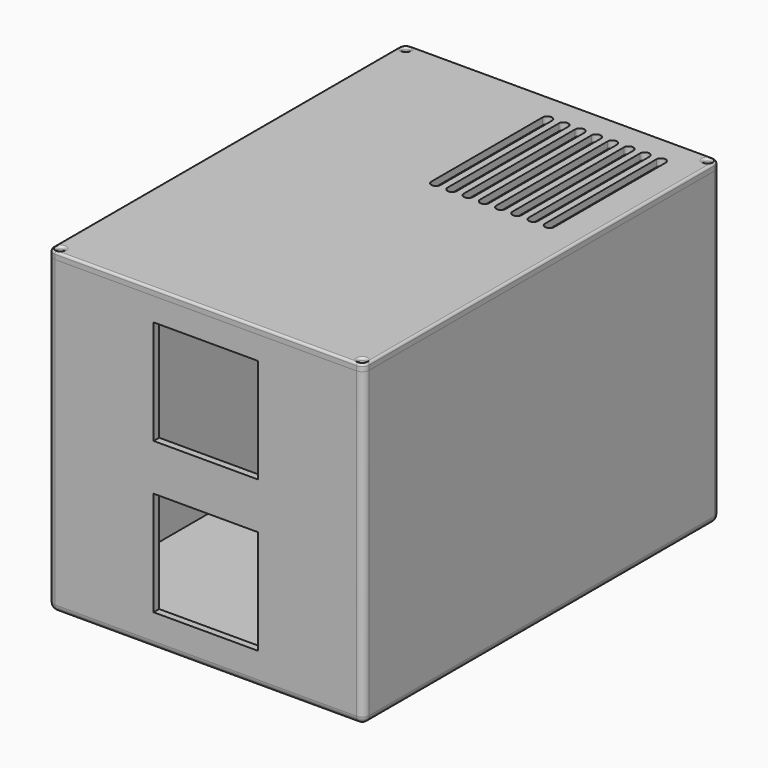
from build123d import *

# Parameters (mm, degrees)
F0_W          = 136
F0_H          = 192
F1_DEPTH      = 4
F2_DEPTH      = 134
F3_W          = 45
F3_H          = 45
F4_DEPTH      = 25
F5_W          = 84
F5_H          = 10
F6_DEPTH      = 20
F8_DEPTH      = 10
F9_W          = 10
F9_H          = 107
F9_R          = 1.5
F10_DEPTH     = 15
F11_R         = 1.5
F12_DEPTH     = 10
F13_W         = 10
F13_H         = 10
F13_W_2       = 27
F13_H_2       = 66
F13_H_3       = 19
F13_R         = 1.6
F14_DEPTH     = 25
F15_W         = 27
F15_H         = 7.5
F16_DEPTH     = 1.5
F17_SIZE      = 1.49999
F18_R         = 3
F19_R         = 3
F20_R         = 3
F22_W         = 65
F22_H         = 125
F22_W_2       = 45
F22_H_2       = 45
F23_DEPTH     = 10
F24_SIZE      = 1
F26_R         = 1.5
F27_DEPTH     = 3
F28_T1_DEPTH  = 186
F28_T3_DEPTH  = 130
F28_T6_ANGLE  = 90
F28_T8_ANGLE  = 90
F28_T10_ANGLE = 90
F28_T12_ANGLE = 90
F30_DEPTH     = 25


# Not quite as in the source:
# - a fillet or chamfer that OpenCascade refuses, or shapes differently, is made with other operations: its cross-section is extruded or revolved along the edge and cut away or added
# - a fillet or chamfer is up to 0.001 mm smaller than in the source, because OpenCascade refuses the exact size


with BuildPart() as f1:
    # F0 (on Top) → F1 (new body)
    with BuildSketch(Plane.XY):
        Rectangle(F0_W, F0_H)
        with BuildLine():
            ThreePointArc((65, -88), (61.4644660941, -89.4644660941), (60, -93))
            Line((60, -93), (-60, -93))
            ThreePointArc((-60, -93), (-61.4644660941, -89.4644660941), (-65, -88))
            Line((-65, -88), (-65, 88))
            ThreePointArc((-65, 88), (-61.4644660941, 89.4644660941), (-60, 93))
            Line((-60, 93), (60, 93))
            ThreePointArc((60, 93), (61.4644660941, 89.4644660941), (65, 88))
            Line((65, 88), (65, -88))
        make_face(mode=Mode.SUBTRACT)
        with BuildLine():
            Line((-60, -93), (60, -93))
            ThreePointArc((60, -93), (61.4644660941, -89.4644660941), (65, -88))
            Line((65, -88), (65, 88))
            ThreePointArc((65, 88), (61.4644660941, 89.4644660941), (60, 93))
            Line((60, 93), (-60, 93))
            ThreePointArc((-60, 93), (-61.4644660941, 89.4644660941), (-65, 88))
            Line((-65, 88), (-65, -88))
            ThreePointArc((-65, -88), (-61.4644660941, -89.4644660941), (-60, -93))
        make_face()
    extrude(amount=F1_DEPTH)

    # F0 (on Top) → F2 (join)
    with BuildSketch(Plane.XY):
        Rectangle(F0_W, F0_H)
        with BuildLine():
            ThreePointArc((65, -88), (61.4644660941, -89.4644660941), (60, -93))
            Line((60, -93), (-60, -93))
            ThreePointArc((-60, -93), (-61.4644660941, -89.4644660941), (-65, -88))
            Line((-65, -88), (-65, 88))
            ThreePointArc((-65, 88), (-61.4644660941, 89.4644660941), (-60, 93))
            Line((-60, 93), (60, 93))
            ThreePointArc((60, 93), (61.4644660941, 89.4644660941), (65, 88))
            Line((65, 88), (65, -88))
        make_face(mode=Mode.SUBTRACT)
    extrude(amount=F2_DEPTH)

    # F3 (on face) → F4 (cut)
    with BuildSketch(Plane.XZ.offset(96)):
        with Locations((0, 101.5)):
            Rectangle(F3_W, F3_H)
        with Locations((0, 36.5)):
            Rectangle(F3_W, F3_H)
    extrude(amount=-F4_DEPTH, mode=Mode.SUBTRACT)

    # F5 (on face) → F6 (join)
    with BuildSketch(Plane.XY.offset(4)):
        with Locations((-23, 78)):
            Rectangle(F5_W, F5_H)
    extrude(amount=F6_DEPTH)

    # F7 (on face) → F8 (cut)
    with BuildSketch(Plane.XZ.offset(-73)):
        Polygon((9, 24), (19, 24), (19, 33.6412377656), (-55, 33.6412377656), (-55, 14), (-28, 14), (-28, 24), (-18, 24), (-18, 14), (9, 14), align=None)
    extrude(amount=-F8_DEPTH, mode=Mode.SUBTRACT)

    # F9 (on face) → F10 (join)
    with BuildSketch(Plane(origin=(65, 0, 0), x_dir=(0, -1, 0), z_dir=(-1, 0, 0))):
        with Locations((-78, 57.5)):
            Rectangle(F9_W, F9_H)
        with Locations((-78, 19)):
            Circle(F9_R, mode=Mode.SUBTRACT)
        with Locations((-78, 106)):
            Circle(F9_R, mode=Mode.SUBTRACT)
        with Locations((-24, 57.5)):
            Rectangle(F9_W, F9_H)
        with Locations((-24, 19)):
            Circle(F9_R, mode=Mode.SUBTRACT)
        with Locations((-24, 106)):
            Circle(F9_R, mode=Mode.SUBTRACT)
    extrude(amount=F10_DEPTH)

    # F11 (on face) → F12 (cut)
    with BuildSketch(Plane.XY.offset(134)):
        with Locations((65, 93)):
            Circle(F11_R)
        with Locations((-65, 93)):
            Circle(F11_R)
        with Locations((65, -93)):
            Circle(F11_R)
        with Locations((-65, -93)):
            Circle(F11_R)
    extrude(amount=-F12_DEPTH, mode=Mode.SUBTRACT)

    # F13 (on face) → F14 (cut)
    with BuildSketch(Plane(origin=(0, 96, 0), x_dir=(-1, 0, 0), z_dir=(0, 1, 0))):
        with Locations((-40, 129)):
            Rectangle(F13_W, F13_H)
        with Locations((41.5, 47)):
            Rectangle(F13_W_2, F13_H_2)
        with Locations((4.5, 47)):
            Rectangle(F13_W_2, F13_H_2)
        with Locations((-24, 26.5)):
            Rectangle(F13_W, F13_H_3)
        with Locations((-24, 14)):
            Circle(F13_R)
        with Locations((-24, 39)):
            Circle(F13_R)
        with Locations((-24, 49)):
            Circle(F13_R)
        with Locations((-24, 61.5)):
            Rectangle(F13_W, F13_H_3)
        with Locations((-24, 74)):
            Circle(F13_R)
    extrude(amount=-F14_DEPTH, mode=Mode.SUBTRACT)

    # F15 (on face) → F16 (cut)
    with BuildSketch(Plane.XZ.offset(-93)):
        with Locations((-41.5, 83.75)):
            Rectangle(F15_W, F15_H)
        with Locations((-4.5, 83.75)):
            Rectangle(F15_W, F15_H)
        with Locations((-41.5, 10.25)):
            Rectangle(F15_W, F15_H)
        with Locations((-4.5, 10.25)):
            Rectangle(F15_W, F15_H)
    extrude(amount=-F16_DEPTH, mode=Mode.SUBTRACT)

    # F17 (size 1.5 in the source; OpenCascade refuses exactly that, so slightly less here)
    f17_edges = [f1.edges().sort_by_distance(p)[0] for p in [
        (-4.5, 94.5, 6.5),
        (-41.5, 94.5, 6.5),
        (-4.5, 94.5, 87.5),
        (-41.5, 94.5, 87.5),
    ]]
    chamfer(f17_edges, length=F17_SIZE)

    # F18
    f18_edges = [f1.edges().sort_by_distance(p)[0] for p in [
        (-68, -96, 67),
        (68, -96, 67),
        (68, 96, 67),
        (-68, 96, 67),
    ]]
    fillet(f18_edges, radius=F18_R)

    # F19
    f19_edges = [f1.edges().sort_by_distance(p)[0] for p in [
        (0, -96, 0),
    ]]
    fillet(f19_edges, radius=F19_R)

    # F20
    f20_edges = [f1.edges().sort_by_distance(p)[0] for p in [
        (45, 94.5, 124),
        (35, 94.5, 124),
    ]]
    fillet(f20_edges, radius=F20_R)


with BuildPart() as f23:
    # F22 (on offset) → F23 (new body)
    with BuildSketch(Plane(origin=(0, -23, 0), x_dir=(-1, 0, 0), z_dir=(0, 1, 0))):
        with Locations((0, 66.5)):
            Rectangle(F22_W, F22_H)
        with Locations((0, 36.5)):
            Rectangle(F22_W_2, F22_H_2, mode=Mode.SUBTRACT)
        with Locations((0, 101.5)):
            Rectangle(F22_W_2, F22_H_2, mode=Mode.SUBTRACT)
    extrude(amount=F23_DEPTH)

    # F24
    f24_edges = [f23.edges().sort_by_distance(p)[0] for p in [
        (-32.5, -23, 66.5),
        (0, -23, 129),
        (32.5, -23, 66.5),
        (0, -23, 4),
        (22.5, -23, 36.5),
        (0, -23, 59),
        (-22.5, -23, 36.5),
        (0, -23, 14),
        (22.5, -23, 101.5),
        (0, -23, 124),
        (-22.5, -23, 101.5),
        (0, -23, 79),
        (-32.5, -13, 66.5),
        (0, -13, 129),
        (32.5, -13, 66.5),
        (0, -13, 4),
        (22.5, -13, 36.5),
        (0, -13, 59),
        (-22.5, -13, 36.5),
        (0, -13, 14),
        (22.5, -13, 101.5),
        (0, -13, 124),
        (-22.5, -13, 101.5),
        (0, -13, 79),
    ]]
    chamfer(f24_edges, length=F24_SIZE)


with BuildPart() as f27:
    # F26 (on offset) → F27 (new body)
    with BuildSketch(Plane.XY.offset(134)):
        with BuildLine():
            ThreePointArc((65, -96), (67.1213203436, -95.1213203436), (68, -93))
            Line((68, -93), (68, 93))
            ThreePointArc((68, 93), (67.1213203436, 95.1213203436), (65, 96))
            Line((65, 96), (-65, 96))
            ThreePointArc((-65, 96), (-67.1213203436, 95.1213203436), (-68, 93))
            Line((-68, 93), (-68, -93))
            ThreePointArc((-68, -93), (-67.1213203436, -95.1213203436), (-65, -96))
            Line((-65, -96), (65, -96))
        make_face()
        with Locations((-65, -93)):
            Circle(F26_R, mode=Mode.SUBTRACT)
        with Locations((65, -93)):
            Circle(F26_R, mode=Mode.SUBTRACT)
        with Locations((-65, 93)):
            Circle(F26_R, mode=Mode.SUBTRACT)
        with BuildLine():
            Line((-60, 93), (60, 93))
            ThreePointArc((60, 93), (61.4644660941, 89.4644660941), (65, 88))
            Line((65, 88), (65, -88))
            ThreePointArc((65, -88), (61.4644660941, -89.4644660941), (60, -93))
            Line((60, -93), (-60, -93))
            ThreePointArc((-60, -93), (-61.4644660941, -89.4644660941), (-65, -88))
            Line((-65, -88), (-65, 88))
            ThreePointArc((-65, 88), (-61.4644660941, 89.4644660941), (-60, 93))
        make_face(mode=Mode.SUBTRACT)
        with Locations((65, 93)):
            Circle(F26_R, mode=Mode.SUBTRACT)
        with BuildLine():
            ThreePointArc((65, 88), (61.4644660941, 89.4644660941), (60, 93))
            Line((60, 93), (-60, 93))
            ThreePointArc((-60, 93), (-61.4644660941, 89.4644660941), (-65, 88))
            Line((-65, 88), (-65, -88))
            ThreePointArc((-65, -88), (-61.4644660941, -89.4644660941), (-60, -93))
            Line((-60, -93), (60, -93))
            ThreePointArc((60, -93), (61.4644660941, -89.4644660941), (65, -88))
            Line((65, -88), (65, 88))
        make_face()
        with BuildLine():
            Line((64, 87.0839202169), (64, -87.0839202169))
            ThreePointArc((64, -87.0839202169), (60.7573593129, -88.7573593129), (59.0839202169, -92))
            Line((59.0839202169, -92), (-59.0839202169, -92))
            ThreePointArc((-59.0839202169, -92), (-60.7573593129, -88.7573593129), (-64, -87.0839202169))
            Line((-64, -87.0839202169), (-64, 87.0839202169))
            ThreePointArc((-64, 87.0839202169), (-60.7573593129, 88.7573593129), (-59.0839202169, 92))
            Line((-59.0839202169, 92), (59.0839202169, 92))
            ThreePointArc((59.0839202169, 92), (60.7573593129, 88.7573593129), (64, 87.0839202169))
        make_face(mode=Mode.SUBTRACT)
        with BuildLine():
            ThreePointArc((59.0839202169, -92), (60.7573593129, -88.7573593129), (64, -87.0839202169))
            Line((64, -87.0839202169), (64, 87.0839202169))
            ThreePointArc((64, 87.0839202169), (60.7573593129, 88.7573593129), (59.0839202169, 92))
            Line((59.0839202169, 92), (-59.0839202169, 92))
            ThreePointArc((-59.0839202169, 92), (-60.7573593129, 88.7573593129), (-64, 87.0839202169))
            Line((-64, 87.0839202169), (-64, -87.0839202169))
            ThreePointArc((-64, -87.0839202169), (-60.7573593129, -88.7573593129), (-59.0839202169, -92))
            Line((-59.0839202169, -92), (59.0839202169, -92))
        make_face()
    extrude(amount=F27_DEPTH)

    # F28: fillet of radius 1 on 12 edges, made by hand

    # F28_s2 → F28_t1 (cut)
    with BuildSketch(Plane.XZ.offset(-93)):
        with BuildLine():
            ThreePointArc((68, 136), (67.7071067812, 136.7071067812), (67, 137))
            Line((67, 137), (68, 137))
            Line((68, 137), (68, 136))
        make_face()
        with BuildLine():
            ThreePointArc((-68, 136), (-67.7071067812, 136.7071067812), (-67, 137))
            Line((-67, 137), (-68, 137))
            Line((-68, 137), (-68, 136))
        make_face()
    extrude(amount=F28_T1_DEPTH, mode=Mode.SUBTRACT)

    # F28_s4 → F28_t3 (cut)
    with BuildSketch(Plane.YZ.offset(-65)):
        with BuildLine():
            ThreePointArc((96, 136), (95.7071067812, 136.7071067812), (95, 137))
            Line((95, 137), (96, 137))
            Line((96, 137), (96, 136))
        make_face()
        with BuildLine():
            ThreePointArc((-96, 136), (-95.7071067812, 136.7071067812), (-95, 137))
            Line((-95, 137), (-96, 137))
            Line((-96, 137), (-96, 136))
        make_face()
    extrude(amount=F28_T3_DEPTH, mode=Mode.SUBTRACT)

    # F28_s5 → F28_t6 (revolve, cut)
    with BuildSketch(Plane.YZ.offset(65)):
        with BuildLine():
            ThreePointArc((-96, 136), (-95.7071067812, 136.7071067812), (-95, 137))
            Line((-95, 137), (-96, 137))
            Line((-96, 137), (-96, 136))
        make_face()
    revolve(axis=Axis((65, -93, 137), (0, 0, 1)), revolution_arc=F28_T6_ANGLE, mode=Mode.SUBTRACT)

    # F28_s7 → F28_t8 (revolve, cut)
    with BuildSketch(Plane.XZ.offset(-93)):
        with BuildLine():
            ThreePointArc((68, 136), (67.7071067812, 136.7071067812), (67, 137))
            Line((67, 137), (68, 137))
            Line((68, 137), (68, 136))
        make_face()
    revolve(axis=Axis((65, 93, 137), (0, 0, 1)), revolution_arc=F28_T8_ANGLE, mode=Mode.SUBTRACT)

    # F28_s9 → F28_t10 (revolve, cut)
    with BuildSketch(Plane.YZ.offset(-65)):
        with BuildLine():
            ThreePointArc((96, 136), (95.7071067812, 136.7071067812), (95, 137))
            Line((95, 137), (96, 137))
            Line((96, 137), (96, 136))
        make_face()
    revolve(axis=Axis((-65, 93, 137), (0, 0, 1)), revolution_arc=F28_T10_ANGLE, mode=Mode.SUBTRACT)

    # F28_s11 → F28_t12 (revolve, cut)
    with BuildSketch(Plane.XZ.offset(93)):
        with BuildLine():
            ThreePointArc((-68, 136), (-67.7071067812, 136.7071067812), (-67, 137))
            Line((-67, 137), (-68, 137))
            Line((-68, 137), (-68, 136))
        make_face()
    revolve(axis=Axis((-65, -93, 137), (0, 0, 1)), revolution_arc=F28_T12_ANGLE, mode=Mode.SUBTRACT)

    # F28_s13 → F28_t14 (revolve, cut)
    with BuildSketch(Plane.XZ.offset(93)):
        with BuildLine():
            ThreePointArc((-63.5, 136), (-63.2071067812, 136.7071067812), (-62.5, 137))
            Line((-62.5, 137), (-63.5, 137))
            Line((-63.5, 137), (-63.5, 136))
        make_face()
    revolve(axis=Axis((-65, -93, 137), (0, 0, 1)), mode=Mode.SUBTRACT)

    # F28_s15 → F28_t16 (revolve, cut)
    with BuildSketch(Plane.XZ.offset(93)):
        with BuildLine():
            ThreePointArc((66.5, 136), (66.7928932188, 136.7071067812), (67.5, 137))
            Line((67.5, 137), (66.5, 137))
            Line((66.5, 137), (66.5, 136))
        make_face()
    revolve(axis=Axis((65, -93, 137), (0, 0, 1)), mode=Mode.SUBTRACT)

    # F28_s17 → F28_t18 (revolve, cut)
    with BuildSketch(Plane.XZ.offset(-93)):
        with BuildLine():
            ThreePointArc((-63.5, 136), (-63.2071067812, 136.7071067812), (-62.5, 137))
            Line((-62.5, 137), (-63.5, 137))
            Line((-63.5, 137), (-63.5, 136))
        make_face()
    revolve(axis=Axis((-65, 93, 137), (0, 0, 1)), mode=Mode.SUBTRACT)

    # F28_s19 → F28_t20 (revolve, cut)
    with BuildSketch(Plane.XZ.offset(-93)):
        with BuildLine():
            ThreePointArc((66.5, 136), (66.7928932188, 136.7071067812), (67.5, 137))
            Line((67.5, 137), (66.5, 137))
            Line((66.5, 137), (66.5, 136))
        make_face()
    revolve(axis=Axis((65, 93, 137), (0, 0, 1)), mode=Mode.SUBTRACT)

    # F29 (on face) → F30 (cut)
    with BuildSketch(Plane.XY.offset(137)):
        with BuildLine():
            ThreePointArc((6, 83), (4, 85), (2, 83))
            Line((2, 83), (2, 23))
            ThreePointArc((2, 23), (4, 21), (6, 23))
            Line((6, 23), (6, 83))
        make_face()
        with BuildLine():
            Line((13, 23), (13, 83))
            ThreePointArc((13, 83), (11, 85), (9, 83))
            Line((9, 83), (9, 23))
            ThreePointArc((9, 23), (11, 21), (13, 23))
        make_face()
        with BuildLine():
            Line((20, 23), (20, 83))
            ThreePointArc((20, 83), (18, 85), (16, 83))
            Line((16, 83), (16, 23))
            ThreePointArc((16, 23), (18, 21), (20, 23))
        make_face()
        with BuildLine():
            Line((27, 23), (27, 83))
            ThreePointArc((27, 83), (25, 85), (23, 83))
            Line((23, 83), (23, 23))
            ThreePointArc((23, 23), (25, 21), (27, 23))
        make_face()
        with BuildLine():
            Line((34, 23), (34, 83))
            ThreePointArc((34, 83), (32, 85), (30, 83))
            Line((30, 83), (30, 23))
            ThreePointArc((30, 23), (32, 21), (34, 23))
        make_face()
        with BuildLine():
            Line((41, 23), (41, 83))
            ThreePointArc((41, 83), (39, 85), (37, 83))
            Line((37, 83), (37, 23))
            ThreePointArc((37, 23), (39, 21), (41, 23))
        make_face()
        with BuildLine():
            Line((48, 23), (48, 83))
            ThreePointArc((48, 83), (46, 85), (44, 83))
            Line((44, 83), (44, 23))
            ThreePointArc((44, 23), (46, 21), (48, 23))
        make_face()
        with BuildLine():
            Line((55, 23), (55, 83))
            ThreePointArc((55, 83), (53, 85), (51, 83))
            Line((51, 83), (51, 23))
            ThreePointArc((51, 23), (53, 21), (55, 23))
        make_face()
    extrude(amount=-F30_DEPTH, mode=Mode.SUBTRACT)


solid = Compound([f1.part, f23.part, f27.part])
